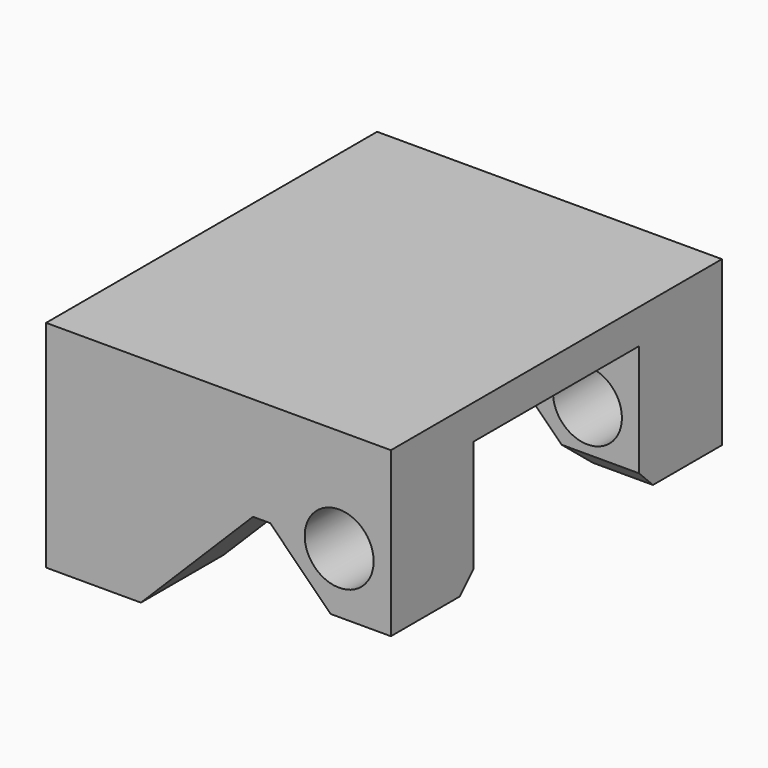
from build123d import *

# Parameters (mm, degrees)
F1_DEPTH      = 170
F1_DEPTH_BACK = 30
F2_R          = 25
F3_DEPTH      = 60
F3_DEPTH_BACK = 60
F5_DEPTH      = 120.001
F5_DEPTH_BACK = 120.001
F6_R          = 20
F7_DEPTH      = 120.001
F7_DEPTH_BACK = 120.001
F8_SIZE       = 10


# Not quite as in the source:
# - a feature names something its author has since deleted; it is built from what else it names


with BuildPart() as f1:
    # F0 (on Right) → F1 (new body, two sides)
    with BuildSketch(Plane.YZ) as f1_sk:
        Polygon((-120, 95), (-120, -30), (-60, -30), (-60, 75), (0, 75), (60, 75), (60, -30), (120, -30), (120, 95), (0, 95), align=None)
    extrude(amount=F1_DEPTH)
    extrude(f1_sk.sketch, amount=-F1_DEPTH_BACK)

    # F2 (on Front) → F3 (join, two sides)
    with BuildSketch(Plane.XZ) as f3_sk:
        Circle(F2_R)
    extrude(amount=F3_DEPTH)
    extrude(f3_sk.sketch, amount=-F3_DEPTH_BACK)

    # F4 (on Front) → F5 (cut, two sides)
    with BuildSketch(Plane.XZ) as f5_sk:
        Polygon((170, -30), (170, 0), (135, 0), (100, 35), (90, 35), (25, -30), align=None)
    extrude(amount=-F5_DEPTH, mode=Mode.SUBTRACT)
    extrude(f5_sk.sketch, amount=F5_DEPTH_BACK, mode=Mode.SUBTRACT)

    # F6 (on Front) → F7 (cut, two sides)
    with BuildSketch(Plane.XZ) as f7_sk:
        with Locations((140, 35)):
            Circle(F6_R)
    extrude(amount=-F7_DEPTH, mode=Mode.SUBTRACT)
    extrude(f7_sk.sketch, amount=F7_DEPTH_BACK, mode=Mode.SUBTRACT)

    # F8
    f8_edges = [f1.edges().sort_by_distance(p)[0] for p in [
        (152.5, -60, 0),
        (152.5, 60, 0),
    ]]
    chamfer(f8_edges, length=F8_SIZE)


solid = f1.part
